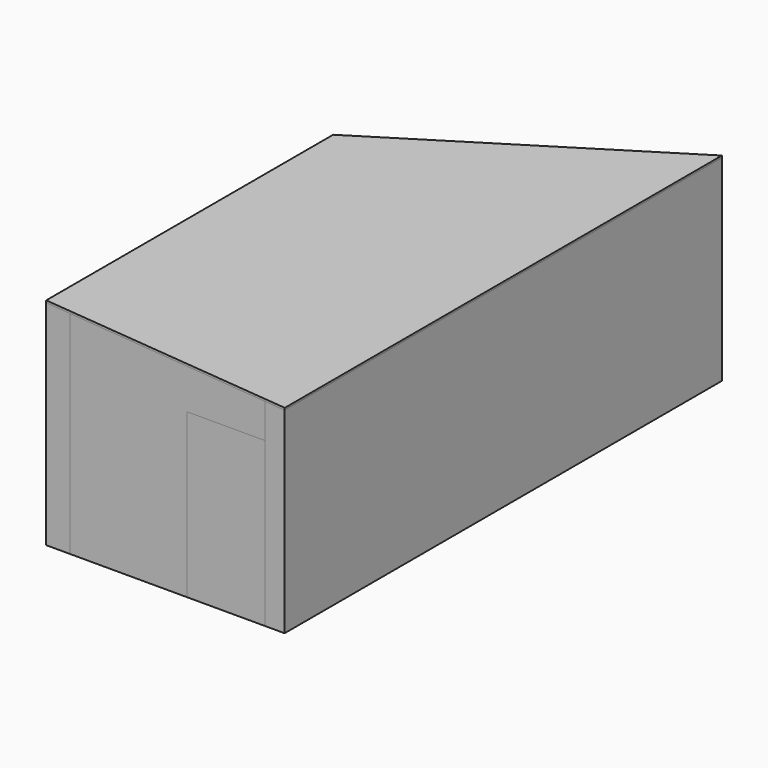
from build123d import *

# Parameters (mm, degrees)
F0_W      = 1397
F0_H      = 2300
F1_DEPTH  = 6400
F3_DEPTH  = 6400
F5_REACH  = 6056.1837849536
F6_T      = -2.5
F9_DEPTH  = 25
F10_REACH = 8727.8551134481
F11_REACH = 8915.8825953498
F7_W      = 914.4
F7_H      = 1912
F12_DEPTH = 100


with BuildPart() as f1:
    # F0 (on Front) → F1 (new body)
    with BuildSketch(Plane.XZ):
        with Locations((-698.5, 1150)):
            Rectangle(F0_W, F0_H)
        with Locations((698.5, 1150)):
            Rectangle(F0_W, F0_H)
    extrude(amount=-F1_DEPTH)

    # F2 (on face) → F3 (join, through all)
    with BuildSketch(Plane(origin=(0, 6400, 0), x_dir=(-1, 0, 0), z_dir=(0, 1, 0))):
        Polygon((-1397, 2300), (1397, 2300), (1397, 2500), align=None)
    extrude(amount=-F3_DEPTH)

    f5_end = f1.faces().sort_by_distance((0, 3200, 2400))[0]
    # F4 (on face) → F5 (cut, up to a face of the model that its end follows)
    with BuildSketch(Plane(origin=(0, 0, 0), x_dir=(1, 0, 0), z_dir=(0, 0, -1))):
        Polygon((1397, -6400), (-1397, -4200), (-1397, -6400), align=None)
    f5_long = extrude(amount=-F5_REACH, mode=Mode.PRIVATE)
    add(split(f5_long, bisect_by=f5_end, keep=Keep.BOTTOM, mode=Mode.PRIVATE), mode=Mode.SUBTRACT)

    # F6
    f6_openings = [f1.faces().sort_by_distance(p)[0] for p in [
        (96.647799, 2688.050314, 0),
    ]]
    offset(amount=F6_T, openings=f6_openings)


with BuildPart() as f9:
    # F8 (on face) → F9 (new body)
    with BuildSketch(Plane(origin=(170.9209123735, 0, 2387.7651458573), x_dir=(0.9974478152, 0, -0.071399271), z_dir=(0.071399271, 0, 0.9974478152))):
        Polygon((1229.2162746817, 0), (1229.2162746817, 6400), (-1571.9327752619, 4200), (-1571.9327752619, 0), align=None)
    extrude(amount=F9_DEPTH)


with BuildPart() as f10:
    f10_end = Plane(origin=(-19.3536070615, 5281.5789575885, 1199.4394861824), x_dir=(-0.7856739006, -0.6186408666, 0), z_dir=(0.6186408666, -0.7856739006, 0))
    # F7 (on face) → F10 (new body, up to a plane its end follows)
    with BuildSketch(Plane.XZ):
        Polygon((1167, 1912), (1167, 0), (1397, 0), (1397, 2300), (1167, 2316.4638511095), align=None)
    f10_long = extrude(amount=-F10_REACH, mode=Mode.PRIVATE)
    add(split(f10_long, bisect_by=f10_end, keep=Keep.TOP, mode=Mode.PRIVATE))


with BuildPart() as f11:
    f11_end = Plane(origin=(-19.3536070615, 5281.5789575885, 1199.4394861824), x_dir=(-0.7856739006, -0.6186408666, 0), z_dir=(0.6186408666, -0.7856739006, 0))
    # F7 (on face) → F11 (new body, up to a plane its end follows)
    with BuildSketch(Plane.XZ):
        Polygon((-1397, 0), (-1114.7586107254, 0), (-1114.7586107254, 1912), (-1114.7586107254, 2479.7966077828), (-1397, 2500), align=None)
    f11_long = extrude(amount=-F11_REACH, mode=Mode.PRIVATE)
    add(split(f11_long, bisect_by=f11_end, keep=Keep.TOP, mode=Mode.PRIVATE))


with BuildPart() as f12:
    # F7 (on face) → F12 (new body)
    with BuildSketch(Plane.XZ):
        with Locations((709.8, 956)):
            Rectangle(F7_W, F7_H)
    extrude(amount=-F12_DEPTH)


solid = Compound([f1.part, f9.part, f10.part, f11.part, f12.part])
